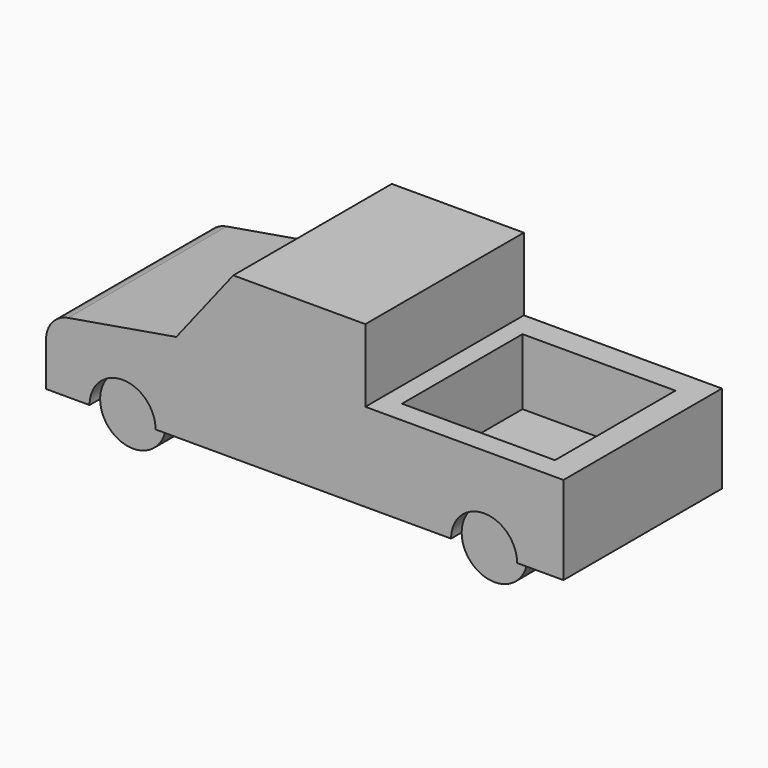
from build123d import *

# Parameters (mm, degrees)
F1_DEPTH  = 19.05
F4_DEPTH  = 19.05
F5_R      = 2.54
F9_DEPTH  = 1.27
F11_DEPTH = 1.27
F13_DEPTH = 1.27
F14_W     = 41.0627422772
F14_H     = 5.3488574922
F15_DEPTH = 22.606
F16_W     = 14.7093571723
F16_H     = 14.4864893518
F17_DEPTH = 6.35


# Not quite as in the source:
# - a feature of the source that left no trace in its solid (it failed there, or was rolled back) is left out


with BuildPart() as f1:
    # F0 (on Front) → F1 (new body)
    with BuildSketch(Plane.XZ):
        Polygon((0, 6.35), (0, 0), (49.7539146826, 0), (49.7539146826, 8.4803946126), (30.7039146826, 8.4803946126), (30.7039146826, 15.4774815776), (18.0039146826, 15.4774815776), (12.5200406866, 8.4803946126), align=None)
    extrude(amount=F1_DEPTH)

    # F2 (on face) + F3 (on face) → F4 (join)
    with BuildSketch(Plane.XZ.offset(19.05)):
        with BuildLine():
            ThreePointArc((4.1796790518, 0), (7.3546790518, -3.175), (10.5296790518, 0))
            Line((10.5296790518, 0), (4.1796790518, 0))
        make_face()
        with BuildLine():
            Line((4.1796790518, 0), (10.5296790518, 0))
            ThreePointArc((10.5296790518, 0), (7.3546790518, 3.175), (4.1796790518, 0))
        make_face()
    with BuildSketch(Plane.XZ.offset(19.05)):
        with BuildLine():
            ThreePointArc((38.9472560108, 0), (42.1222560108, -3.175), (45.2972560108, 0))
            Line((45.2972560108, 0), (38.9472560108, 0))
        make_face()
    extrude(amount=-F4_DEPTH)

    # F5
    f5_edges = [f1.edges().sort_by_distance(p)[0] for p in [
        (0, -9.525, 6.35),
    ]]
    fillet(f5_edges, radius=F5_R)

    # F8 (on face) → F9 (cut)
    with BuildSketch(Plane(origin=(0, 0, 0), x_dir=(-1, 0, 0), z_dir=(0, 1, 0))):
        with BuildLine():
            ThreePointArc((-10.5296790518, 0), (-7.3546790518, -3.175), (-4.1796790518, 0))
            ThreePointArc((-4.1796790518, 0), (-7.3546790518, 3.175), (-10.5296790518, 0))
        make_face()
    extrude(amount=-F9_DEPTH, mode=Mode.SUBTRACT)

    # F10 (on face) → F11 (cut)
    with BuildSketch(Plane(origin=(0, 0, 0), x_dir=(-1, 0, 0), z_dir=(0, 1, 0))):
        with BuildLine():
            ThreePointArc((-45.2972560108, 0), (-42.1222560108, -3.175), (-38.9472560108, 0))
            ThreePointArc((-38.9472560108, 0), (-42.1222560108, 3.175), (-45.2972560108, 0))
        make_face()
    extrude(amount=-F11_DEPTH, mode=Mode.SUBTRACT)

    # F12 (on face) → F13 (cut)
    with BuildSketch(Plane.XZ.offset(19.05)):
        with BuildLine():
            ThreePointArc((38.9472560108, 0), (42.1222560108, -3.175), (45.2972560108, 0))
            ThreePointArc((45.2972560108, 0), (42.1222560108, 3.175), (38.9472560108, 0))
        make_face()
        with BuildLine():
            ThreePointArc((4.1796790518, 0), (7.3546790518, -3.175), (10.5296790518, 0))
            ThreePointArc((10.5296790518, 0), (7.3546790518, 3.175), (4.1796790518, 0))
        make_face()
    extrude(amount=-F13_DEPTH, mode=Mode.SUBTRACT)

    # F14 (on face) → F15 (cut)
    with BuildSketch(Plane(origin=(0, 0, 0), x_dir=(1, 0, 0), z_dir=(0, 0, -1))):
        with Locations((24.7110501904, 9.5833707601)):
            Rectangle(F14_W, F14_H)
    extrude(amount=F15_DEPTH, mode=Mode.SUBTRACT)

    # F16 (on face) → F17 (cut)
    with BuildSketch(Plane.XY.offset(8.4803946126)):
        with Locations((39.8935656995, -9.6948046703)):
            Rectangle(F16_W, F16_H)
    extrude(amount=-F17_DEPTH, mode=Mode.SUBTRACT)


solid = f1.part
